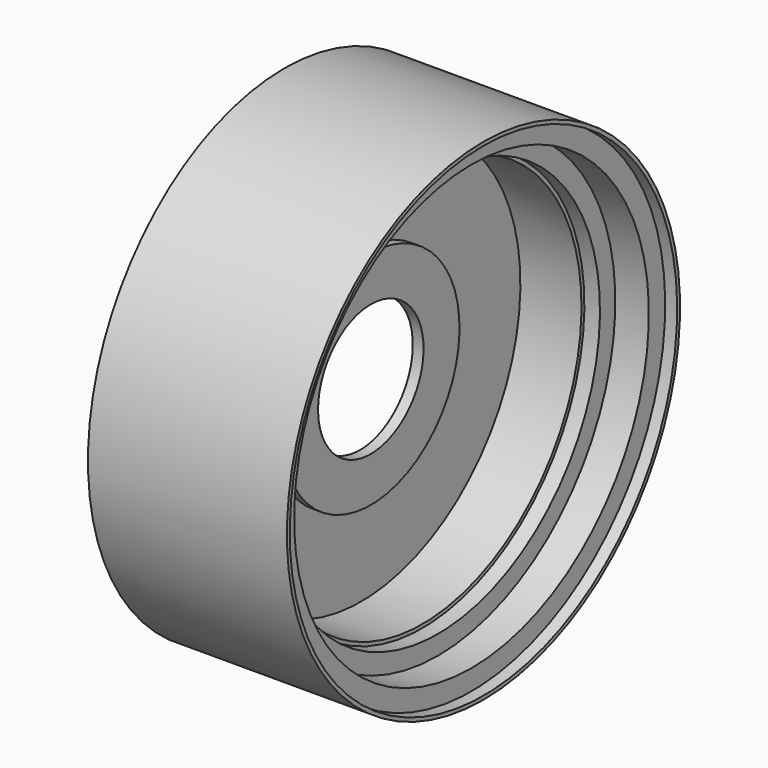
from build123d import *

# Parameters (mm, degrees)
F2_R            = 6
F3_DEPTH        = 6
F3_COPIES_COUNT = 4


# Not quite as in the source:
# - a pattern or mirror of a feature is missing from the dataset's text; its kind, count and spacing are read off the source's solid


with BuildPart() as f1:
    # F0 (on Front) → F1 (revolve)
    with BuildSketch(Plane.XZ):
        Polygon((166, 205), (0, 205), (0, 202), (10, 202), (10, 185), (38, 185), (38, 169), (61, 169), (61, 87.5), (63, 87.5), (63, 55), (72, 55), (72, 92.5), (64, 92.5), (64, 166), (115, 166), (115, 169), (128, 169), (128, 185), (156, 185), (156, 202), (166, 202), align=None)
    revolve(axis=Axis((83, 0, 0), (1, 0, 0)))

    # F2 (on face) → F3 (cut)
    with BuildSketch(Plane(origin=(63, 0, 0), x_dir=(0, -1, 0), z_dir=(-1, 0, 0))):
        with Locations((0, 66)):
            Circle(F2_R)
    f3 = extrude(amount=-F3_DEPTH, mode=Mode.SUBTRACT)

    # F3_copies: F3 ×4 about axis
    f3_copies_axis = Axis((0, 0, 0), (1, 0, 0))
    for i in range(1, F3_COPIES_COUNT):
        add(f3.rotate(f3_copies_axis, i * 360 / F3_COPIES_COUNT), mode=Mode.SUBTRACT)


solid = f1.part
